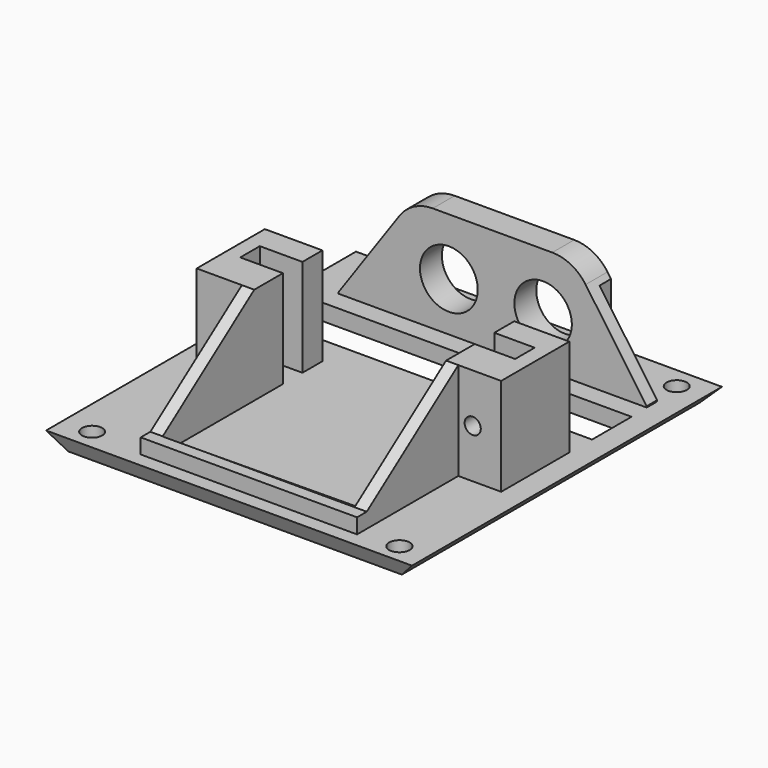
from build123d import *

# Parameters (mm, degrees)
F0_W         = 44.9817739427
F0_H         = 49.7469753027
F3_DEPTH     = 2
F4_DEPTH     = 12
F2_W         = 37.9821762908
F2_H         = 6.06366992
F5_DEPTH     = 6.6
F6_DEPTH     = 13
F7_R         = 3.5309507028
F7_R_2       = 3.55
F8_DEPTH     = 5
F9_SIZE2     = 12.8533320607
F9_SIZE      = 9
F10_R        = 5
F11_R        = 0.9934278603
F12_DEPTH    = 11
F13_R        = 0.9970874125
F14_DEPTH    = 11
F15_R        = 1.25
F15_R_2      = 1.261860196
F16_DEPTH    = 4
F18_DEPTH    = 29.1
F19_SIZE     = 1.99999
F20_T1_DEPTH = 63.2072532601


# Not quite as in the source:
# - a fillet or chamfer that OpenCascade refuses, or shapes differently, is made with other operations: its cross-section is extruded or revolved along the edge and cut away or added
# - a fillet or chamfer is up to 0.001 mm smaller than in the source, because OpenCascade refuses the exact size


with BuildPart() as f3:
    # F0 (on Top) → F3 (new body)
    with BuildSketch(Plane.XY):
        with Locations((-22.4908869714, 24.8734876513)):
            Rectangle(F0_W, F0_H)
    extrude(amount=-F3_DEPTH)

    # F1 (on face) → F4 (join)
    with BuildSketch(Plane.XY):
        Polygon((-9.6775945276, 22.7995335534), (-9.6775945276, 4.4446666725), (-33.2585461438, 4.2995335534), (-33.2585461438, 22.7995335534), (-38.4990237653, 22.7995335534), (-38.4990237653, 25.7995335534), (-33.2585461438, 25.7995335534), (-33.2585461438, 28.8677942008), (-40.3328314424, 28.8677942008), (-40.3328314424, 18.3987934142), (-34.7744636238, 18.3987934142), (-34.7744636238, 2.8445292264), (-8.1775945276, 2.8445292264), (-8.1775945276, 18.3987934142), (-2.9087525018, 18.3987934142), (-2.9087525018, 28.8677942008), (-9.6775945276, 28.8677942008), (-9.6775945276, 25.7995335534), (-4.7087525018, 25.7995335534), (-4.7087525018, 22.7995335534), align=None)
    extrude(amount=F4_DEPTH)

    # F2 (on Top) → F5 (cut)
    with BuildSketch(Plane.XY):
        with Locations((-21.8701980775, 35.3616550565)):
            Rectangle(F2_W, F2_H)
    extrude(amount=-F5_DEPTH, mode=Mode.SUBTRACT)

    # F1 (on face) → F6 (join)
    with BuildSketch(Plane.XY):
        Polygon((-40.8417806029, 42.3996723965), (-40.8417806029, 40.7995335534), (-2.9438226484, 40.7995335534), (-2.9438226484, 42.3996723965), (-10.0181093439, 42.3996723965), (-10.0181093439, 44.1682427898), (-33.2621894777, 44.1682427898), (-33.2621894777, 42.3996723965), align=None)
    extrude(amount=F6_DEPTH)

    # F7 (on face) → F8 (cut)
    with BuildSketch(Plane(origin=(0, 44.1682427898, 0), x_dir=(-1, 0, 0), z_dir=(0, 1, 0))):
        with Locations((15.6775945276, 6)):
            Circle(F7_R)
        with Locations((27.2585461438, 6)):
            Circle(F7_R_2)
    extrude(amount=-F8_DEPTH, mode=Mode.SUBTRACT)

    # F9
    f9_edges = [f3.edges().sort_by_distance(p)[0] for p in [
        (-40.841781, 41.599603, 13),
        (-2.943823, 41.599603, 13),
    ]]
    f9_side = f3.faces().sort_by_distance((-21.790726, 42.280107, 13))[0]
    chamfer(f9_edges, length=F9_SIZE, length2=F9_SIZE2, reference=f9_side)

    # F10
    f10_edges = [f3.edges().sort_by_distance(p)[0] for p in [
        (-11.943823, 42.483888, 13),
        (-31.841781, 42.483888, 13),
    ]]
    fillet(f10_edges, radius=F10_R)

    # F11 (on face) → F12 (cut)
    with BuildSketch(Plane(origin=(0, 28.8677942008, 0), x_dir=(-1, 0, 0), z_dir=(0, 1, 0))):
        with Locations((6.41001435, 6)):
            Circle(F11_R)
    extrude(amount=-F12_DEPTH, mode=Mode.SUBTRACT)

    # F13 (on face) → F14 (cut)
    with BuildSketch(Plane(origin=(0, 28.8677942008, 0), x_dir=(-1, 0, 0), z_dir=(0, 1, 0))):
        with Locations((36.6457030177, 6)):
            Circle(F13_R)
    extrude(amount=-F14_DEPTH, mode=Mode.SUBTRACT)

    # F15 (on face) → F16 (cut)
    with BuildSketch(Plane(origin=(0, 0, -2), x_dir=(1, 0, 0), z_dir=(0, 0, -1))):
        with Locations((-41.3694195449, -3.6203172058)):
            Circle(F15_R)
        with Locations((-3.4651088063, -3.4644450061)):
            Circle(F15_R_2)
        with Locations((-41.3694195449, -46.0678450763)):
            Circle(F15_R)
        with Locations((-3.4651088063, -46.0678450763)):
            Circle(F15_R)
    extrude(amount=-F16_DEPTH, mode=Mode.SUBTRACT)

    # F17 (on face) → F18 (cut)
    with BuildSketch(Plane(origin=(-34.7744636238, 0, 0), x_dir=(0, -1, 0), z_dir=(-1, 0, 0))):
        Polygon((-2.8445292264, 12), (-18.3987934142, 12), (-4.3348377745, 1.8491647206), (-2.8445292264, 1.8491647206), align=None)
    extrude(amount=-F18_DEPTH, mode=Mode.SUBTRACT)

    # F19 (size 2 in the source; OpenCascade refuses exactly that, so slightly less here)
    f19_edges = [f3.edges().sort_by_distance(p)[0] for p in [
        (-44.981774, 24.873488, -2),
        (0, 24.873488, -2),
    ]]
    chamfer(f19_edges, length=F19_SIZE)

    # F20: chamfer of 2 x 4.289013841 on 2 edges, made by hand

    # F20_s2 → F20_t1 (cut)
    with BuildSketch(Plane.YZ.offset(-54.0945136014)):
        Polygon((2, -2), (0, 2.289013841), (0, -2), align=None)
        Polygon((47.7469753027, -2), (49.7469753027, 2.289013841), (49.7469753027, -2), align=None)
    extrude(amount=F20_T1_DEPTH, mode=Mode.SUBTRACT)


solid = f3.part
